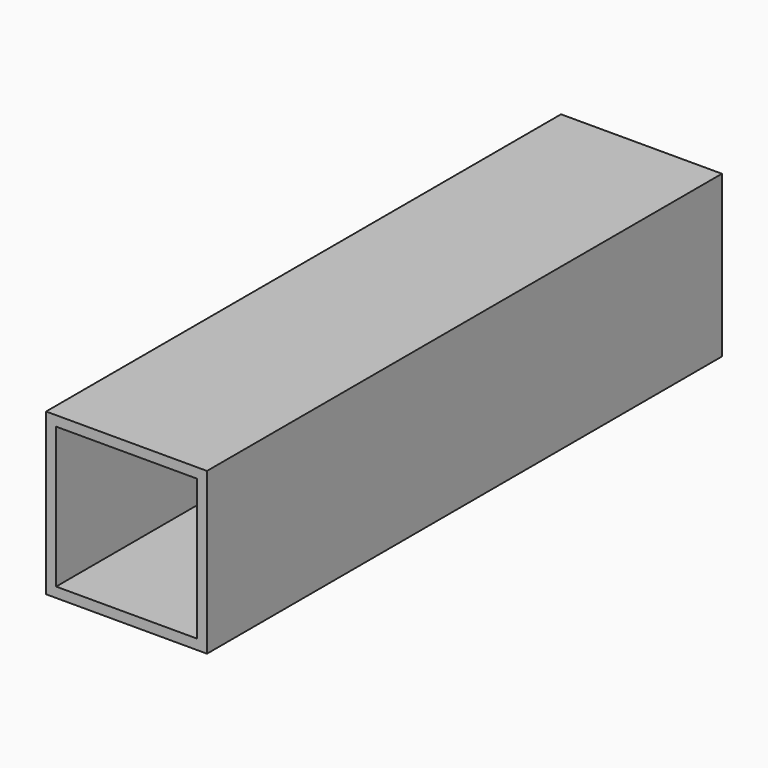
from build123d import *

# Parameters (mm, degrees)
F1_W     = 25.4
F1_H     = 25.4
F1_W_2   = 22.225
F1_H_2   = 22.225
F2_DEPTH = 101.6


# Not quite as in the source:
# - a variable given as a bare number and used for a length is read in inches; the dataset says mm whatever the document's units were


with BuildPart() as f2:
    # F1 (on Front) → F2 (new body)
    with BuildSketch(Plane.XZ):
        Rectangle(F1_W, F1_H)
        Rectangle(F1_W_2, F1_H_2, mode=Mode.SUBTRACT)
    extrude(amount=F2_DEPTH)


solid = f2.part
